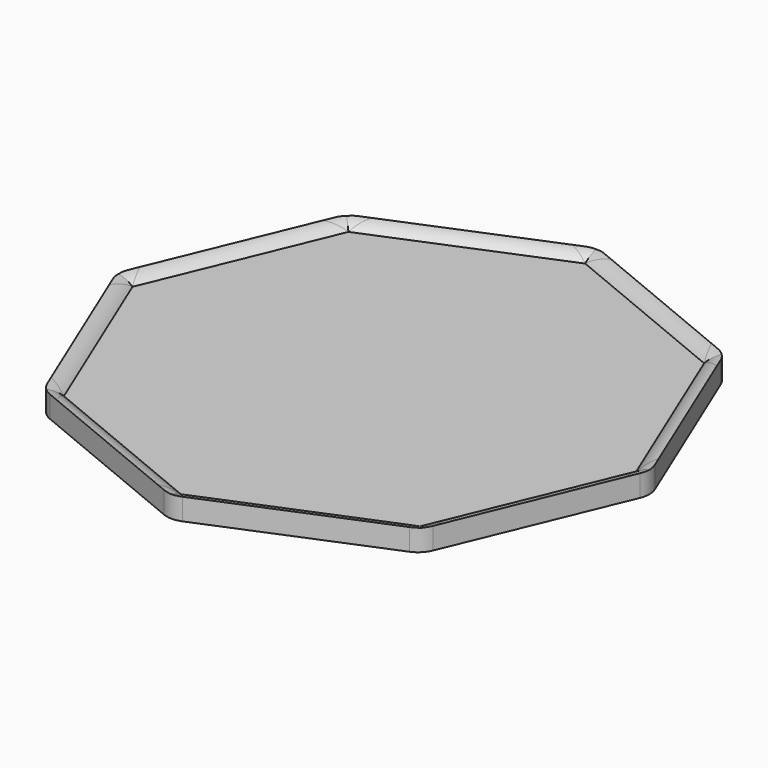
from build123d import *

# Parameters (mm, degrees)
F1_DEPTH      = 3
F3_DEPTH      = 1.5
F4_T1_DEPTH   = 14.8553390593
F4_T6_DEPTH   = 57.4552821399
F4_T12_DEPTH  = 57.4552821399
F4_T18_DEPTH  = 57.4552821399
F4_T24_DEPTH  = 57.4552821399
F4_T30_DEPTH  = 57.4552821399
F4_T36_DEPTH  = 57.4552821399
F4_T42_DEPTH  = 57.4552821399
F4_T48_DEPTH  = 57.4552821399
F4_T55_DEPTH  = 57.4552821399
F4_T61_DEPTH  = 57.4552821399
F4_T70_DEPTH  = 57.4552821399
F4_T76_DEPTH  = 57.4552821399
F4_T85_DEPTH  = 57.4552821399
F4_T91_DEPTH  = 57.4552821399
F4_T100_DEPTH = 57.4552821399
F4_T106_DEPTH = 57.4552821399
F4_T115_DEPTH = 57.4552821399
F4_T121_DEPTH = 57.4552821399
F4_T130_DEPTH = 57.4552821399
F4_T136_DEPTH = 57.4552821399
F4_T145_DEPTH = 57.4552821399
F4_T151_DEPTH = 57.4552821399
F4_T160_DEPTH = 57.4552821399
F4_T166_DEPTH = 57.4552821399


# Not quite as in the source:
# - a fillet or chamfer that OpenCascade refuses, or shapes differently, is made with other operations: its cross-section is extruded or revolved along the edge and cut away or added


with BuildPart() as f1:
    # F0 (on Top) → F1 (new body)
    with BuildSketch(Plane.XY):
        Polygon((38.8908729653, 38.8908729653), (0, 55), (-38.8908729653, 38.8908729653), (-55, 0), (-38.8908729653, -38.8908729653), (0, -55), (38.8908729653, -38.8908729653), (55, 0), align=None)
    extrude(amount=F1_DEPTH)

    # F2 (on face) → F3 (join)
    with BuildSketch(Plane.XY.offset(3)):
        Polygon((0, 55), (-38.8908729653, 38.8908729653), (-55, 0), (-38.8908729653, -38.8908729653), (0, -55), (38.8908729653, -38.8908729653), (55, 0), (38.8908729653, 38.8908729653), align=None)
        Polygon((-36.5872103086, 36.5872103086), (0, 51.7421290278), (36.5872103086, 36.5872103086), (51.7421290278, 0), (36.5872103086, -36.5872103086), (0, -51.7421290278), (-36.5872103086, -36.5872103086), (-51.7421290278, 0), align=None, mode=Mode.SUBTRACT)
    extrude(amount=F3_DEPTH)

    # F4: fillet of radius 5 on 16 edges, made by hand

    # F4_s2 → F4_t1 (cut)
    with BuildSketch(Plane.XY.offset(-5.1776695297)):
        with BuildLine():
            ThreePointArc((-1.9134171618, -54.2074366611), (0, -54.5880389985), (1.9134171618, -54.2074366611))
            Line((1.9134171618, -54.2074366611), (0, -55))
            Line((0, -55), (-1.9134171618, -54.2074366611))
        make_face()
        with BuildLine():
            ThreePointArc((39.6834363042, -36.9774558034), (38.5995725475, -38.5995725475), (36.9774558034, -39.6834363042))
            Line((36.9774558034, -39.6834363042), (38.8908729653, -38.8908729653))
            Line((38.8908729653, -38.8908729653), (39.6834363042, -36.9774558034))
        make_face()
        with BuildLine():
            ThreePointArc((-36.9774558034, -39.6834363042), (-38.5995725475, -38.5995725475), (-39.6834363042, -36.9774558034))
            Line((-39.6834363042, -36.9774558034), (-38.8908729653, -38.8908729653))
            Line((-38.8908729653, -38.8908729653), (-36.9774558034, -39.6834363042))
        make_face()
        with BuildLine():
            ThreePointArc((-54.2074366611, -1.9134171618), (-54.5880389985, 0), (-54.2074366611, 1.9134171618))
            Line((-54.2074366611, 1.9134171618), (-55, 0))
            Line((-55, 0), (-54.2074366611, -1.9134171618))
        make_face()
        with BuildLine():
            ThreePointArc((54.2074366611, -1.9134171618), (54.5880389985, 0), (54.2074366611, 1.9134171618))
            Line((54.2074366611, 1.9134171618), (55, 0))
            Line((55, 0), (54.2074366611, -1.9134171618))
        make_face()
        with BuildLine():
            ThreePointArc((36.9774558034, 39.6834363042), (38.5995725475, 38.5995725475), (39.6834363042, 36.9774558034))
            Line((39.6834363042, 36.9774558034), (38.8908729653, 38.8908729653))
            Line((38.8908729653, 38.8908729653), (36.9774558034, 39.6834363042))
        make_face()
        with BuildLine():
            ThreePointArc((-1.9134171618, 54.2074366611), (0, 54.5880389985), (1.9134171618, 54.2074366611))
            Line((1.9134171618, 54.2074366611), (0, 55))
            Line((0, 55), (-1.9134171618, 54.2074366611))
        make_face()
        with BuildLine():
            ThreePointArc((-39.6834363042, 36.9774558034), (-38.5995725475, 38.5995725475), (-36.9774558034, 39.6834363042))
            Line((-36.9774558034, 39.6834363042), (-38.8908729653, 38.8908729653))
            Line((-38.8908729653, 38.8908729653), (-39.6834363042, 36.9774558034))
        make_face()
    extrude(amount=F4_T1_DEPTH, mode=Mode.SUBTRACT)


with BuildPart() as f4_tool4:
    # F4_s5 → F4_t6 (new body)
    with BuildSketch(Plane(origin=(-26.5408796018, -10.9935922884, 0), x_dir=(0, 0, 1), z_dir=(0.9238795325, 0.3826834324, 0))):
        with BuildLine():
            ThreePointArc((4.5, -51.3742081917), (4.1097722286, -49.4377165186), (3, -47.8034939774))
            Line((3, -47.8034939774), (4.5, -47.8034939774))
            Line((4.5, -47.8034939774), (4.5, -51.3742081917))
        make_face()
    extrude(amount=F4_T6_DEPTH)

    split(bisect_by=Plane(origin=(18.2936051543, 44.1646696682, 0), x_dir=(0, 0, 1), z_dir=(-0.3826834324, -0.9238795325, 0)), keep=Keep.TOP)

    split(bisect_by=Plane(origin=(-44.1646696682, 18.2936051543, 0), x_dir=(0, 0, 1), z_dir=(0.9238795325, -0.3826834324, 0)), keep=Keep.TOP)


with BuildPart() as f1_1:
    add(f1.part)

    # F4_t3: cut F4_tool4
    add(f4_tool4.part, mode=Mode.SUBTRACT)


with BuildPart() as f4_tool10:
    # F4_s11 → F4_t12 (new body)
    with BuildSketch(Plane(origin=(-10.9935922884, -26.5408796018, 0), x_dir=(0, 0, 1), z_dir=(0.3826834324, 0.9238795325, 0))):
        with BuildLine():
            ThreePointArc((4.5, -51.3742081917), (4.1097722286, -49.4377165186), (3, -47.8034939774))
            Line((3, -47.8034939774), (4.5, -47.8034939774))
            Line((4.5, -47.8034939774), (4.5, -51.3742081917))
        make_face()
    extrude(amount=F4_T12_DEPTH)

    split(bisect_by=Plane(origin=(-44.1646696682, -18.2936051543, 0), x_dir=(0, 0, 1), z_dir=(0.9238795325, 0.3826834324, 0)), keep=Keep.TOP)

    split(bisect_by=Plane(origin=(-18.2936051543, 44.1646696682, 0), x_dir=(0, 0, 1), z_dir=(0.3826834324, -0.9238795325, 0)), keep=Keep.TOP)


with BuildPart() as f1_2:
    add(f1_1.part)

    # F4_t9: cut F4_tool10
    add(f4_tool10.part, mode=Mode.SUBTRACT)


with BuildPart() as f4_tool16:
    # F4_s17 → F4_t18 (new body)
    with BuildSketch(Plane(origin=(-26.5408796018, 10.9935922884, 0), x_dir=(0, 0, 1), z_dir=(0.9238795325, -0.3826834324, 0))):
        with BuildLine():
            ThreePointArc((4.5, -51.3742081917), (4.1097722286, -49.4377165186), (3, -47.8034939774))
            Line((3, -47.8034939774), (4.5, -47.8034939774))
            Line((4.5, -47.8034939774), (4.5, -51.3742081917))
        make_face()
    extrude(amount=F4_T18_DEPTH)

    split(bisect_by=Plane(origin=(44.1646696682, 18.2936051543, 0), x_dir=(0, 0, 1), z_dir=(-0.9238795325, -0.3826834324, 0)), keep=Keep.TOP)

    split(bisect_by=Plane(origin=(-18.2936051543, 44.1646696682, 0), x_dir=(0, 0, 1), z_dir=(0.3826834324, -0.9238795325, 0)), keep=Keep.TOP)


with BuildPart() as f1_3:
    add(f1_2.part)

    # F4_t15: cut F4_tool16
    add(f4_tool16.part, mode=Mode.SUBTRACT)


with BuildPart() as f4_tool22:
    # F4_s23 → F4_t24 (new body)
    with BuildSketch(Plane(origin=(-10.9935922884, 26.5408796018, 0), x_dir=(0, 0, 1), z_dir=(0.3826834324, -0.9238795325, 0))):
        with BuildLine():
            ThreePointArc((4.5, -51.3742081917), (4.1097722286, -49.4377165186), (3, -47.8034939774))
            Line((3, -47.8034939774), (4.5, -47.8034939774))
            Line((4.5, -47.8034939774), (4.5, -51.3742081917))
        make_face()
    extrude(amount=F4_T24_DEPTH)

    split(bisect_by=Plane(origin=(44.1646696682, -18.2936051543, 0), x_dir=(0, 0, 1), z_dir=(-0.9238795325, 0.3826834324, 0)), keep=Keep.TOP)

    split(bisect_by=Plane(origin=(18.2936051543, 44.1646696682, 0), x_dir=(0, 0, 1), z_dir=(-0.3826834324, -0.9238795325, 0)), keep=Keep.TOP)


with BuildPart() as f1_4:
    add(f1_3.part)

    # F4_t21: cut F4_tool22
    add(f4_tool22.part, mode=Mode.SUBTRACT)


with BuildPart() as f4_tool28:
    # F4_s29 → F4_t30 (new body)
    with BuildSketch(Plane(origin=(10.9935922884, 26.5408796018, 0), x_dir=(0, 0, 1), z_dir=(-0.3826834324, -0.9238795325, 0))):
        with BuildLine():
            ThreePointArc((4.5, -51.3742081917), (4.1097722286, -49.4377165186), (3, -47.8034939774))
            Line((3, -47.8034939774), (4.5, -47.8034939774))
            Line((4.5, -47.8034939774), (4.5, -51.3742081917))
        make_face()
    extrude(amount=F4_T30_DEPTH)

    split(bisect_by=Plane(origin=(18.2936051543, -44.1646696682, 0), x_dir=(0, 0, 1), z_dir=(-0.3826834324, 0.9238795325, 0)), keep=Keep.TOP)

    split(bisect_by=Plane(origin=(44.1646696682, 18.2936051543, 0), x_dir=(0, 0, 1), z_dir=(-0.9238795325, -0.3826834324, 0)), keep=Keep.TOP)


with BuildPart() as f1_5:
    add(f1_4.part)

    # F4_t27: cut F4_tool28
    add(f4_tool28.part, mode=Mode.SUBTRACT)


with BuildPart() as f4_tool34:
    # F4_s35 → F4_t36 (new body)
    with BuildSketch(Plane(origin=(26.5408796018, 10.9935922884, 0), x_dir=(0, 0, 1), z_dir=(-0.9238795325, -0.3826834324, 0))):
        with BuildLine():
            ThreePointArc((4.5, -51.3742081917), (4.1097722286, -49.4377165186), (3, -47.8034939774))
            Line((3, -47.8034939774), (4.5, -47.8034939774))
            Line((4.5, -47.8034939774), (4.5, -51.3742081917))
        make_face()
    extrude(amount=F4_T36_DEPTH)

    split(bisect_by=Plane(origin=(-18.2936051543, -44.1646696682, 0), x_dir=(0, 0, 1), z_dir=(0.3826834324, 0.9238795325, 0)), keep=Keep.TOP)

    split(bisect_by=Plane(origin=(44.1646696682, -18.2936051543, 0), x_dir=(0, 0, 1), z_dir=(-0.9238795325, 0.3826834324, 0)), keep=Keep.TOP)


with BuildPart() as f1_6:
    add(f1_5.part)

    # F4_t33: cut F4_tool34
    add(f4_tool34.part, mode=Mode.SUBTRACT)


with BuildPart() as f4_tool40:
    # F4_s41 → F4_t42 (new body)
    with BuildSketch(Plane(origin=(10.9935922884, -26.5408796018, 0), x_dir=(0, 0, 1), z_dir=(-0.3826834324, 0.9238795325, 0))):
        with BuildLine():
            ThreePointArc((4.5, -51.3742081917), (4.1097722286, -49.4377165186), (3, -47.8034939774))
            Line((3, -47.8034939774), (4.5, -47.8034939774))
            Line((4.5, -47.8034939774), (4.5, -51.3742081917))
        make_face()
    extrude(amount=F4_T42_DEPTH)

    split(bisect_by=Plane(origin=(-18.2936051543, -44.1646696682, 0), x_dir=(0, 0, 1), z_dir=(0.3826834324, 0.9238795325, 0)), keep=Keep.TOP)

    split(bisect_by=Plane(origin=(-44.1646696682, 18.2936051543, 0), x_dir=(0, 0, 1), z_dir=(0.9238795325, -0.3826834324, 0)), keep=Keep.TOP)


with BuildPart() as f1_7:
    add(f1_6.part)

    # F4_t39: cut F4_tool40
    add(f4_tool40.part, mode=Mode.SUBTRACT)


with BuildPart() as f4_tool46:
    # F4_s47 → F4_t48 (new body)
    with BuildSketch(Plane(origin=(26.5408796018, -10.9935922884, 0), x_dir=(0, 0, 1), z_dir=(-0.9238795325, 0.3826834324, 0))):
        with BuildLine():
            ThreePointArc((4.5, -51.3742081917), (4.1097722286, -49.4377165186), (3, -47.8034939774))
            Line((3, -47.8034939774), (4.5, -47.8034939774))
            Line((4.5, -47.8034939774), (4.5, -51.3742081917))
        make_face()
    extrude(amount=F4_T48_DEPTH)

    split(bisect_by=Plane(origin=(-44.1646696682, -18.2936051543, 0), x_dir=(0, 0, 1), z_dir=(0.9238795325, 0.3826834324, 0)), keep=Keep.TOP)

    split(bisect_by=Plane(origin=(18.2936051543, -44.1646696682, 0), x_dir=(0, 0, 1), z_dir=(-0.3826834324, 0.9238795325, 0)), keep=Keep.TOP)


with BuildPart() as f1_8:
    add(f1_7.part)

    # F4_t45: cut F4_tool46
    add(f4_tool46.part, mode=Mode.SUBTRACT)


with BuildPart() as f4_tool53:
    # F4_s54 → F4_t55 (new body)
    with BuildSketch(Plane(origin=(-10.9935922884, -26.5408796018, 0), x_dir=(0, 0, 1), z_dir=(0.3826834324, 0.9238795325, 0))):
        with BuildLine():
            ThreePointArc((4.5, -51.3742081917), (4.1097722286, -49.4377165186), (3, -47.8034939774))
            Line((3, -47.8034939774), (4.5, -47.8034939774))
            Line((4.5, -47.8034939774), (4.5, -51.3742081917))
        make_face()
    extrude(amount=F4_T55_DEPTH)

    split(bisect_by=Plane(origin=(-46.9454364826, 19.4454364826, 0), x_dir=(0, 0, 1), z_dir=(0.9238795325, -0.3826834324, 0)), keep=Keep.TOP)

    split(bisect_by=Plane(origin=(-19.4454364826, 46.9454364826, 0), x_dir=(0, 0, 1), z_dir=(0.3826834324, -0.9238795325, 0)), keep=Keep.TOP)

    split(bisect_by=Plane(origin=(-18.2936051543, 44.1646696682, 0), x_dir=(0, 0, 1), z_dir=(-0.3826834324, 0.9238795325, 0)), keep=Keep.TOP)


with BuildPart() as f4_tool59:
    # F4_s60 → F4_t61 (new body)
    with BuildSketch(Plane(origin=(-26.5408796018, -10.9935922884, 0), x_dir=(0, 0, 1), z_dir=(0.9238795325, 0.3826834324, 0))):
        with BuildLine():
            ThreePointArc((4.5, -51.3742081917), (4.1097722286, -49.4377165186), (3, -47.8034939774))
            Line((3, -47.8034939774), (4.5, -47.8034939774))
            Line((4.5, -47.8034939774), (4.5, -51.3742081917))
        make_face()
    extrude(amount=F4_T61_DEPTH)

    split(bisect_by=Plane(origin=(-46.9454364826, 19.4454364826, 0), x_dir=(0, 0, 1), z_dir=(0.9238795325, -0.3826834324, 0)), keep=Keep.TOP)

    split(bisect_by=Plane(origin=(-19.4454364826, 46.9454364826, 0), x_dir=(0, 0, 1), z_dir=(0.3826834324, -0.9238795325, 0)), keep=Keep.TOP)

    split(bisect_by=Plane(origin=(-44.1646696682, 18.2936051543, 0), x_dir=(0, 0, 1), z_dir=(-0.9238795325, 0.3826834324, 0)), keep=Keep.TOP)


with BuildPart() as f4_tool53_1:
    add(f4_tool53.part)

    # F4_t65: intersect F4_tool59
    add(f4_tool59.part, mode=Mode.INTERSECT)


with BuildPart() as f1_9:
    add(f1_8.part)

    # F4_t51: cut F4_tool53
    add(f4_tool53_1.part, mode=Mode.SUBTRACT)


with BuildPart() as f4_tool68:
    # F4_s69 → F4_t70 (new body)
    with BuildSketch(Plane(origin=(-26.5408796018, -10.9935922884, 0), x_dir=(0, 0, 1), z_dir=(0.9238795325, 0.3826834324, 0))):
        with BuildLine():
            ThreePointArc((4.5, -51.3742081917), (4.1097722286, -49.4377165186), (3, -47.8034939774))
            Line((3, -47.8034939774), (4.5, -47.8034939774))
            Line((4.5, -47.8034939774), (4.5, -51.3742081917))
        make_face()
    extrude(amount=F4_T70_DEPTH)

    split(bisect_by=Plane(origin=(-19.4454364826, 46.9454364826, 0), x_dir=(0, 0, 1), z_dir=(0.3826834324, -0.9238795325, 0)), keep=Keep.TOP)

    split(bisect_by=Plane(origin=(19.4454364826, 46.9454364826, 0), x_dir=(0, 0, 1), z_dir=(-0.3826834324, -0.9238795325, 0)), keep=Keep.TOP)

    split(bisect_by=Plane(origin=(18.2936051543, 44.1646696682, 0), x_dir=(0, 0, 1), z_dir=(0.3826834324, 0.9238795325, 0)), keep=Keep.TOP)


with BuildPart() as f4_tool74:
    # F4_s75 → F4_t76 (new body)
    with BuildSketch(Plane(origin=(-26.5408796018, 10.9935922884, 0), x_dir=(0, 0, 1), z_dir=(0.9238795325, -0.3826834324, 0))):
        with BuildLine():
            ThreePointArc((4.5, -51.3742081917), (4.1097722286, -49.4377165186), (3, -47.8034939774))
            Line((3, -47.8034939774), (4.5, -47.8034939774))
            Line((4.5, -47.8034939774), (4.5, -51.3742081917))
        make_face()
    extrude(amount=F4_T76_DEPTH)

    split(bisect_by=Plane(origin=(-19.4454364826, 46.9454364826, 0), x_dir=(0, 0, 1), z_dir=(0.3826834324, -0.9238795325, 0)), keep=Keep.TOP)

    split(bisect_by=Plane(origin=(19.4454364826, 46.9454364826, 0), x_dir=(0, 0, 1), z_dir=(-0.3826834324, -0.9238795325, 0)), keep=Keep.TOP)

    split(bisect_by=Plane(origin=(-18.2936051543, 44.1646696682, 0), x_dir=(0, 0, 1), z_dir=(-0.3826834324, 0.9238795325, 0)), keep=Keep.TOP)


with BuildPart() as f4_tool68_1:
    add(f4_tool68.part)

    # F4_t80: intersect F4_tool74
    add(f4_tool74.part, mode=Mode.INTERSECT)


with BuildPart() as f1_10:
    add(f1_9.part)

    # F4_t66: cut F4_tool68
    add(f4_tool68_1.part, mode=Mode.SUBTRACT)


with BuildPart() as f4_tool83:
    # F4_s84 → F4_t85 (new body)
    with BuildSketch(Plane(origin=(-10.9935922884, -26.5408796018, 0), x_dir=(0, 0, 1), z_dir=(0.3826834324, 0.9238795325, 0))):
        with BuildLine():
            ThreePointArc((4.5, -51.3742081917), (4.1097722286, -49.4377165186), (3, -47.8034939774))
            Line((3, -47.8034939774), (4.5, -47.8034939774))
            Line((4.5, -47.8034939774), (4.5, -51.3742081917))
        make_face()
    extrude(amount=F4_T85_DEPTH)

    split(bisect_by=Plane(origin=(-46.9454364826, -19.4454364826, 0), x_dir=(0, 0, 1), z_dir=(0.9238795325, 0.3826834324, 0)), keep=Keep.TOP)

    split(bisect_by=Plane(origin=(-46.9454364826, 19.4454364826, 0), x_dir=(0, 0, 1), z_dir=(0.9238795325, -0.3826834324, 0)), keep=Keep.TOP)

    split(bisect_by=Plane(origin=(-44.1646696682, -18.2936051543, 0), x_dir=(0, 0, 1), z_dir=(-0.9238795325, -0.3826834324, 0)), keep=Keep.TOP)


with BuildPart() as f4_tool89:
    # F4_s90 → F4_t91 (new body)
    with BuildSketch(Plane(origin=(10.9935922884, -26.5408796018, 0), x_dir=(0, 0, 1), z_dir=(-0.3826834324, 0.9238795325, 0))):
        with BuildLine():
            ThreePointArc((4.5, -51.3742081917), (4.1097722286, -49.4377165186), (3, -47.8034939774))
            Line((3, -47.8034939774), (4.5, -47.8034939774))
            Line((4.5, -47.8034939774), (4.5, -51.3742081917))
        make_face()
    extrude(amount=F4_T91_DEPTH)

    split(bisect_by=Plane(origin=(-46.9454364826, -19.4454364826, 0), x_dir=(0, 0, 1), z_dir=(0.9238795325, 0.3826834324, 0)), keep=Keep.TOP)

    split(bisect_by=Plane(origin=(-46.9454364826, 19.4454364826, 0), x_dir=(0, 0, 1), z_dir=(0.9238795325, -0.3826834324, 0)), keep=Keep.TOP)

    split(bisect_by=Plane(origin=(-44.1646696682, 18.2936051543, 0), x_dir=(0, 0, 1), z_dir=(-0.9238795325, 0.3826834324, 0)), keep=Keep.TOP)


with BuildPart() as f4_tool83_1:
    add(f4_tool83.part)

    # F4_t95: intersect F4_tool89
    add(f4_tool89.part, mode=Mode.INTERSECT)


with BuildPart() as f1_11:
    add(f1_10.part)

    # F4_t81: cut F4_tool83
    add(f4_tool83_1.part, mode=Mode.SUBTRACT)


with BuildPart() as f4_tool98:
    # F4_s99 → F4_t100 (new body)
    with BuildSketch(Plane(origin=(-26.5408796018, 10.9935922884, 0), x_dir=(0, 0, 1), z_dir=(0.9238795325, -0.3826834324, 0))):
        with BuildLine():
            ThreePointArc((4.5, -51.3742081917), (4.1097722286, -49.4377165186), (3, -47.8034939774))
            Line((3, -47.8034939774), (4.5, -47.8034939774))
            Line((4.5, -47.8034939774), (4.5, -51.3742081917))
        make_face()
    extrude(amount=F4_T100_DEPTH)

    split(bisect_by=Plane(origin=(19.4454364826, 46.9454364826, 0), x_dir=(0, 0, 1), z_dir=(-0.3826834324, -0.9238795325, 0)), keep=Keep.TOP)

    split(bisect_by=Plane(origin=(46.9454364826, 19.4454364826, 0), x_dir=(0, 0, 1), z_dir=(-0.9238795325, -0.3826834324, 0)), keep=Keep.TOP)

    split(bisect_by=Plane(origin=(44.1646696682, 18.2936051543, 0), x_dir=(0, 0, 1), z_dir=(0.9238795325, 0.3826834324, 0)), keep=Keep.TOP)


with BuildPart() as f4_tool104:
    # F4_s105 → F4_t106 (new body)
    with BuildSketch(Plane(origin=(-10.9935922884, 26.5408796018, 0), x_dir=(0, 0, 1), z_dir=(0.3826834324, -0.9238795325, 0))):
        with BuildLine():
            ThreePointArc((4.5, -51.3742081917), (4.1097722286, -49.4377165186), (3, -47.8034939774))
            Line((3, -47.8034939774), (4.5, -47.8034939774))
            Line((4.5, -47.8034939774), (4.5, -51.3742081917))
        make_face()
    extrude(amount=F4_T106_DEPTH)

    split(bisect_by=Plane(origin=(19.4454364826, 46.9454364826, 0), x_dir=(0, 0, 1), z_dir=(-0.3826834324, -0.9238795325, 0)), keep=Keep.TOP)

    split(bisect_by=Plane(origin=(46.9454364826, 19.4454364826, 0), x_dir=(0, 0, 1), z_dir=(-0.9238795325, -0.3826834324, 0)), keep=Keep.TOP)

    split(bisect_by=Plane(origin=(18.2936051543, 44.1646696682, 0), x_dir=(0, 0, 1), z_dir=(0.3826834324, 0.9238795325, 0)), keep=Keep.TOP)


with BuildPart() as f4_tool98_1:
    add(f4_tool98.part)

    # F4_t110: intersect F4_tool104
    add(f4_tool104.part, mode=Mode.INTERSECT)


with BuildPart() as f1_12:
    add(f1_11.part)

    # F4_t96: cut F4_tool98
    add(f4_tool98_1.part, mode=Mode.SUBTRACT)


with BuildPart() as f4_tool113:
    # F4_s114 → F4_t115 (new body)
    with BuildSketch(Plane(origin=(-10.9935922884, 26.5408796018, 0), x_dir=(0, 0, 1), z_dir=(0.3826834324, -0.9238795325, 0))):
        with BuildLine():
            ThreePointArc((4.5, -51.3742081917), (4.1097722286, -49.4377165186), (3, -47.8034939774))
            Line((3, -47.8034939774), (4.5, -47.8034939774))
            Line((4.5, -47.8034939774), (4.5, -51.3742081917))
        make_face()
    extrude(amount=F4_T115_DEPTH)

    split(bisect_by=Plane(origin=(46.9454364826, -19.4454364826, 0), x_dir=(0, 0, 1), z_dir=(-0.9238795325, 0.3826834324, 0)), keep=Keep.TOP)

    split(bisect_by=Plane(origin=(46.9454364826, 19.4454364826, 0), x_dir=(0, 0, 1), z_dir=(-0.9238795325, -0.3826834324, 0)), keep=Keep.TOP)

    split(bisect_by=Plane(origin=(44.1646696682, -18.2936051543, 0), x_dir=(0, 0, 1), z_dir=(0.9238795325, -0.3826834324, 0)), keep=Keep.TOP)


with BuildPart() as f4_tool119:
    # F4_s120 → F4_t121 (new body)
    with BuildSketch(Plane(origin=(10.9935922884, 26.5408796018, 0), x_dir=(0, 0, 1), z_dir=(-0.3826834324, -0.9238795325, 0))):
        with BuildLine():
            ThreePointArc((4.5, -51.3742081917), (4.1097722286, -49.4377165186), (3, -47.8034939774))
            Line((3, -47.8034939774), (4.5, -47.8034939774))
            Line((4.5, -47.8034939774), (4.5, -51.3742081917))
        make_face()
    extrude(amount=F4_T121_DEPTH)

    split(bisect_by=Plane(origin=(46.9454364826, -19.4454364826, 0), x_dir=(0, 0, 1), z_dir=(-0.9238795325, 0.3826834324, 0)), keep=Keep.TOP)

    split(bisect_by=Plane(origin=(46.9454364826, 19.4454364826, 0), x_dir=(0, 0, 1), z_dir=(-0.9238795325, -0.3826834324, 0)), keep=Keep.TOP)

    split(bisect_by=Plane(origin=(44.1646696682, 18.2936051543, 0), x_dir=(0, 0, 1), z_dir=(0.9238795325, 0.3826834324, 0)), keep=Keep.TOP)


with BuildPart() as f4_tool113_1:
    add(f4_tool113.part)

    # F4_t125: intersect F4_tool119
    add(f4_tool119.part, mode=Mode.INTERSECT)


with BuildPart() as f1_13:
    add(f1_12.part)

    # F4_t111: cut F4_tool113
    add(f4_tool113_1.part, mode=Mode.SUBTRACT)


with BuildPart() as f4_tool128:
    # F4_s129 → F4_t130 (new body)
    with BuildSketch(Plane(origin=(10.9935922884, 26.5408796018, 0), x_dir=(0, 0, 1), z_dir=(-0.3826834324, -0.9238795325, 0))):
        with BuildLine():
            ThreePointArc((4.5, -51.3742081917), (4.1097722286, -49.4377165186), (3, -47.8034939774))
            Line((3, -47.8034939774), (4.5, -47.8034939774))
            Line((4.5, -47.8034939774), (4.5, -51.3742081917))
        make_face()
    extrude(amount=F4_T130_DEPTH)

    split(bisect_by=Plane(origin=(46.9454364826, -19.4454364826, 0), x_dir=(0, 0, 1), z_dir=(-0.9238795325, 0.3826834324, 0)), keep=Keep.TOP)

    split(bisect_by=Plane(origin=(18.2936051543, -44.1646696682, 0), x_dir=(0, 0, 1), z_dir=(0.3826834324, -0.9238795325, 0)), keep=Keep.TOP)

    split(bisect_by=Plane(origin=(19.4454364826, -46.9454364826, 0), x_dir=(0, 0, 1), z_dir=(-0.3826834324, 0.9238795325, 0)), keep=Keep.TOP)


with BuildPart() as f4_tool134:
    # F4_s135 → F4_t136 (new body)
    with BuildSketch(Plane(origin=(26.5408796018, 10.9935922884, 0), x_dir=(0, 0, 1), z_dir=(-0.9238795325, -0.3826834324, 0))):
        with BuildLine():
            ThreePointArc((4.5, -51.3742081917), (4.1097722286, -49.4377165186), (3, -47.8034939774))
            Line((3, -47.8034939774), (4.5, -47.8034939774))
            Line((4.5, -47.8034939774), (4.5, -51.3742081917))
        make_face()
    extrude(amount=F4_T136_DEPTH)

    split(bisect_by=Plane(origin=(46.9454364826, -19.4454364826, 0), x_dir=(0, 0, 1), z_dir=(-0.9238795325, 0.3826834324, 0)), keep=Keep.TOP)

    split(bisect_by=Plane(origin=(44.1646696682, -18.2936051543, 0), x_dir=(0, 0, 1), z_dir=(0.9238795325, -0.3826834324, 0)), keep=Keep.TOP)

    split(bisect_by=Plane(origin=(19.4454364826, -46.9454364826, 0), x_dir=(0, 0, 1), z_dir=(-0.3826834324, 0.9238795325, 0)), keep=Keep.TOP)


with BuildPart() as f4_tool128_1:
    add(f4_tool128.part)

    # F4_t140: intersect F4_tool134
    add(f4_tool134.part, mode=Mode.INTERSECT)


with BuildPart() as f1_14:
    add(f1_13.part)

    # F4_t126: cut F4_tool128
    add(f4_tool128_1.part, mode=Mode.SUBTRACT)


with BuildPart() as f4_tool143:
    # F4_s144 → F4_t145 (new body)
    with BuildSketch(Plane(origin=(26.5408796018, 10.9935922884, 0), x_dir=(0, 0, 1), z_dir=(-0.9238795325, -0.3826834324, 0))):
        with BuildLine():
            ThreePointArc((4.5, -51.3742081917), (4.1097722286, -49.4377165186), (3, -47.8034939774))
            Line((3, -47.8034939774), (4.5, -47.8034939774))
            Line((4.5, -47.8034939774), (4.5, -51.3742081917))
        make_face()
    extrude(amount=F4_T145_DEPTH)

    split(bisect_by=Plane(origin=(-19.4454364826, -46.9454364826, 0), x_dir=(0, 0, 1), z_dir=(0.3826834324, 0.9238795325, 0)), keep=Keep.TOP)

    split(bisect_by=Plane(origin=(-18.2936051543, -44.1646696682, 0), x_dir=(0, 0, 1), z_dir=(-0.3826834324, -0.9238795325, 0)), keep=Keep.TOP)

    split(bisect_by=Plane(origin=(19.4454364826, -46.9454364826, 0), x_dir=(0, 0, 1), z_dir=(-0.3826834324, 0.9238795325, 0)), keep=Keep.TOP)


with BuildPart() as f4_tool149:
    # F4_s150 → F4_t151 (new body)
    with BuildSketch(Plane(origin=(26.5408796018, -10.9935922884, 0), x_dir=(0, 0, 1), z_dir=(-0.9238795325, 0.3826834324, 0))):
        with BuildLine():
            ThreePointArc((4.5, -51.3742081917), (4.1097722286, -49.4377165186), (3, -47.8034939774))
            Line((3, -47.8034939774), (4.5, -47.8034939774))
            Line((4.5, -47.8034939774), (4.5, -51.3742081917))
        make_face()
    extrude(amount=F4_T151_DEPTH)

    split(bisect_by=Plane(origin=(-19.4454364826, -46.9454364826, 0), x_dir=(0, 0, 1), z_dir=(0.3826834324, 0.9238795325, 0)), keep=Keep.TOP)

    split(bisect_by=Plane(origin=(18.2936051543, -44.1646696682, 0), x_dir=(0, 0, 1), z_dir=(0.3826834324, -0.9238795325, 0)), keep=Keep.TOP)

    split(bisect_by=Plane(origin=(19.4454364826, -46.9454364826, 0), x_dir=(0, 0, 1), z_dir=(-0.3826834324, 0.9238795325, 0)), keep=Keep.TOP)


with BuildPart() as f4_tool143_1:
    add(f4_tool143.part)

    # F4_t155: intersect F4_tool149
    add(f4_tool149.part, mode=Mode.INTERSECT)


with BuildPart() as f1_15:
    add(f1_14.part)

    # F4_t141: cut F4_tool143
    add(f4_tool143_1.part, mode=Mode.SUBTRACT)


with BuildPart() as f4_tool158:
    # F4_s159 → F4_t160 (new body)
    with BuildSketch(Plane(origin=(26.5408796018, -10.9935922884, 0), x_dir=(0, 0, 1), z_dir=(-0.9238795325, 0.3826834324, 0))):
        with BuildLine():
            ThreePointArc((4.5, -51.3742081917), (4.1097722286, -49.4377165186), (3, -47.8034939774))
            Line((3, -47.8034939774), (4.5, -47.8034939774))
            Line((4.5, -47.8034939774), (4.5, -51.3742081917))
        make_face()
    extrude(amount=F4_T160_DEPTH)

    split(bisect_by=Plane(origin=(-19.4454364826, -46.9454364826, 0), x_dir=(0, 0, 1), z_dir=(0.3826834324, 0.9238795325, 0)), keep=Keep.TOP)

    split(bisect_by=Plane(origin=(-46.9454364826, -19.4454364826, 0), x_dir=(0, 0, 1), z_dir=(0.9238795325, 0.3826834324, 0)), keep=Keep.TOP)

    split(bisect_by=Plane(origin=(-44.1646696682, -18.2936051543, 0), x_dir=(0, 0, 1), z_dir=(-0.9238795325, -0.3826834324, 0)), keep=Keep.TOP)


with BuildPart() as f4_tool164:
    # F4_s165 → F4_t166 (new body)
    with BuildSketch(Plane(origin=(10.9935922884, -26.5408796018, 0), x_dir=(0, 0, 1), z_dir=(-0.3826834324, 0.9238795325, 0))):
        with BuildLine():
            ThreePointArc((4.5, -51.3742081917), (4.1097722286, -49.4377165186), (3, -47.8034939774))
            Line((3, -47.8034939774), (4.5, -47.8034939774))
            Line((4.5, -47.8034939774), (4.5, -51.3742081917))
        make_face()
    extrude(amount=F4_T166_DEPTH)

    split(bisect_by=Plane(origin=(-19.4454364826, -46.9454364826, 0), x_dir=(0, 0, 1), z_dir=(0.3826834324, 0.9238795325, 0)), keep=Keep.TOP)

    split(bisect_by=Plane(origin=(-46.9454364826, -19.4454364826, 0), x_dir=(0, 0, 1), z_dir=(0.9238795325, 0.3826834324, 0)), keep=Keep.TOP)

    split(bisect_by=Plane(origin=(-18.2936051543, -44.1646696682, 0), x_dir=(0, 0, 1), z_dir=(-0.3826834324, -0.9238795325, 0)), keep=Keep.TOP)


with BuildPart() as f4_tool158_1:
    add(f4_tool158.part)

    # F4_t170: intersect F4_tool164
    add(f4_tool164.part, mode=Mode.INTERSECT)


with BuildPart() as f1_16:
    add(f1_15.part)

    # F4_t156: cut F4_tool158
    add(f4_tool158_1.part, mode=Mode.SUBTRACT)


solid = f1_16.part
